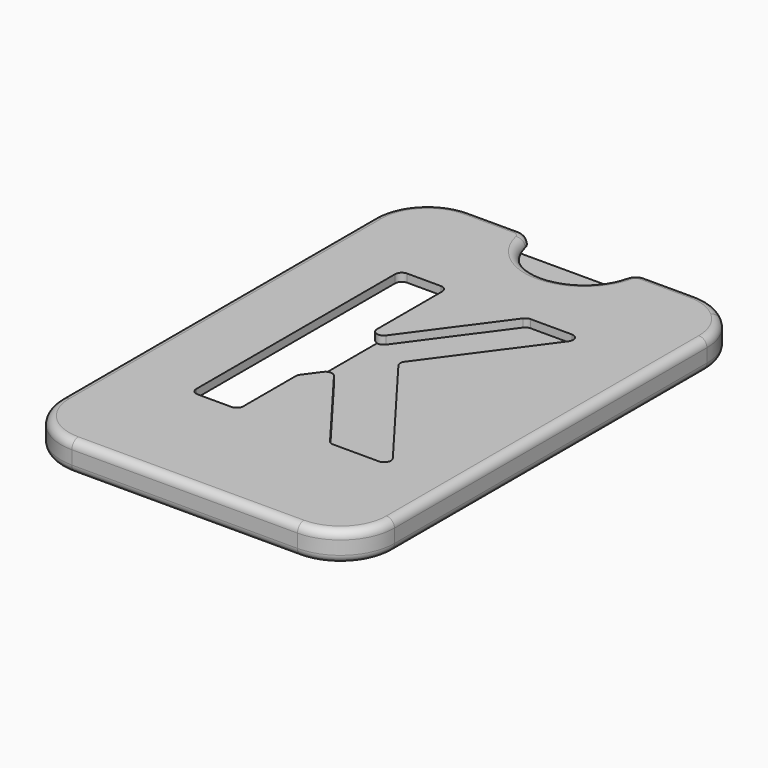
from build123d import *

# Parameters (mm, degrees)
F1_DEPTH = 2.794
F2_DEPTH = 1.27
F4_DEPTH = 2.54
F6_DEPTH = 2.54
F8_DEPTH = 2.54
F9_R     = 2.54
F10_R    = 1.52399
F11_R    = 1.27
F12_R    = 1.26999


# Not quite as in the source:
# - a fillet or chamfer is up to 0.001 mm smaller than in the source, because OpenCascade refuses the exact size


with BuildPart() as f1:
    # F0 (on Top) → F1 (new body, symmetric)
    with BuildSketch(Plane.XY):
        with BuildLine():
            Line((13.4556421247, 40.506048555), (-29.0893578753, 40.506048555))
            ThreePointArc((-29.0893578753, 40.506048555), (-32.6881934203, 39.8473107196), (-35.8203578753, 37.9565175945))
            Line((-35.8203578753, 37.9565175945), (-35.8203578753, 30.346048555))
            ThreePointArc((-35.8203578753, 30.346048555), (-33.8488936195, 35.1055842992), (-29.0893578753, 37.077048555))
            Line((-29.0893578753, 37.077048555), (13.4556421247, 37.077048555))
            ThreePointArc((13.4556421247, 37.077048555), (18.2151778689, 35.1055842992), (20.1866421247, 30.346048555))
            Line((20.1866421247, 30.346048555), (20.1866421247, 37.9565175945))
            ThreePointArc((20.1866421247, 37.9565175945), (17.0544776697, 39.8473107196), (13.4556421247, 40.506048555))
        make_face()
        with BuildLine():
            ThreePointArc((-29.0893578753, 37.077048555), (-33.8488936195, 35.1055842992), (-35.8203578753, 30.346048555))
            Line((-35.8203578753, 30.346048555), (-35.8203578753, -43.313951445))
            ThreePointArc((-35.8203578753, -43.313951445), (-33.8488936195, -48.0734871891), (-29.0893578753, -50.044951445))
            Line((-29.0893578753, -50.044951445), (13.4556421247, -50.044951445))
            ThreePointArc((13.4556421247, -50.044951445), (18.2151778689, -48.0734871891), (20.1866421247, -43.313951445))
            Line((20.1866421247, -43.313951445), (20.1866421247, 30.346048555))
            ThreePointArc((20.1866421247, 30.346048555), (18.2151778689, 35.1055842992), (13.4556421247, 37.077048555))
            Line((13.4556421247, 37.077048555), (-29.0893578753, 37.077048555))
        make_face()
        with BuildLine():
            Line((-35.8203578753, 30.346048555), (-35.8203578753, 37.9565175945))
            ThreePointArc((-35.8203578753, 37.9565175945), (-38.3525257999, 34.5196944432), (-39.2493578753, 30.346048555))
            Line((-39.2493578753, 30.346048555), (-39.2493578753, -43.313951445))
            ThreePointArc((-39.2493578753, -43.313951445), (-36.2735627721, -50.4981563418), (-29.0893578753, -53.473951445))
            Line((-29.0893578753, -53.473951445), (13.4556421247, -53.473951445))
            ThreePointArc((13.4556421247, -53.473951445), (20.6398470216, -50.4981563418), (23.6156421247, -43.313951445))
            Line((23.6156421247, -43.313951445), (23.6156421247, 30.346048555))
            ThreePointArc((23.6156421247, 30.346048555), (22.7188100493, 34.5196944432), (20.1866421247, 37.9565175945))
            Line((20.1866421247, 37.9565175945), (20.1866421247, 30.346048555))
            Line((20.1866421247, 30.346048555), (20.1866421247, -43.313951445))
            ThreePointArc((20.1866421247, -43.313951445), (18.2151778689, -48.0734871891), (13.4556421247, -50.044951445))
            Line((13.4556421247, -50.044951445), (-29.0893578753, -50.044951445))
            ThreePointArc((-29.0893578753, -50.044951445), (-33.8488936195, -48.0734871891), (-35.8203578753, -43.313951445))
            Line((-35.8203578753, -43.313951445), (-35.8203578753, 30.346048555))
        make_face()
    extrude(amount=F1_DEPTH, both=True)

    # F0 (on Top) → F2 (cut, symmetric)
    with BuildSketch(Plane.XY):
        with BuildLine():
            Line((13.4556421247, 40.506048555), (-29.0893578753, 40.506048555))
            ThreePointArc((-29.0893578753, 40.506048555), (-32.6881934203, 39.8473107196), (-35.8203578753, 37.9565175945))
            Line((-35.8203578753, 37.9565175945), (-35.8203578753, 30.346048555))
            ThreePointArc((-35.8203578753, 30.346048555), (-33.8488936195, 35.1055842992), (-29.0893578753, 37.077048555))
            Line((-29.0893578753, 37.077048555), (13.4556421247, 37.077048555))
            ThreePointArc((13.4556421247, 37.077048555), (18.2151778689, 35.1055842992), (20.1866421247, 30.346048555))
            Line((20.1866421247, 30.346048555), (20.1866421247, 37.9565175945))
            ThreePointArc((20.1866421247, 37.9565175945), (17.0544776697, 39.8473107196), (13.4556421247, 40.506048555))
        make_face()
        with BuildLine():
            ThreePointArc((-29.0893578753, 37.077048555), (-33.8488936195, 35.1055842992), (-35.8203578753, 30.346048555))
            Line((-35.8203578753, 30.346048555), (-35.8203578753, -43.313951445))
            ThreePointArc((-35.8203578753, -43.313951445), (-33.8488936195, -48.0734871891), (-29.0893578753, -50.044951445))
            Line((-29.0893578753, -50.044951445), (13.4556421247, -50.044951445))
            ThreePointArc((13.4556421247, -50.044951445), (18.2151778689, -48.0734871891), (20.1866421247, -43.313951445))
            Line((20.1866421247, -43.313951445), (20.1866421247, 30.346048555))
            ThreePointArc((20.1866421247, 30.346048555), (18.2151778689, 35.1055842992), (13.4556421247, 37.077048555))
            Line((13.4556421247, 37.077048555), (-29.0893578753, 37.077048555))
        make_face()
    extrude(amount=F2_DEPTH, both=True, mode=Mode.SUBTRACT)

    # F3 (on face) → F4 (cut)
    with BuildSketch(Plane.XY.offset(2.794)):
        Polygon((-16.199497506, 18.9658571035), (-25.0740814954, 18.9658571035), (-25.0740814954, -30.413236469), (-16.199497506, -30.413236469), (-16.199497506, -16.4083634515), (-12.8775097826, -11.8783802343), (1.1254162528, -30.413236469), (12.8968711942, -30.413236469), (-7.0793794499, -3.9718389452), (9.7415978089, 18.9658571035), (-1.1809705757, 18.9658571035), (-16.199497506, -1.5139521565), align=None)
    extrude(amount=-F4_DEPTH, mode=Mode.SUBTRACT)

    # F5 (on face) → F6 (cut)
    with BuildSketch(Plane(origin=(0, 0, -2.794), x_dir=(1, 0, 0), z_dir=(0, 0, -1))):
        with BuildLine():
            Line((-29.1631240398, 40.1679472998), (-29.1631240398, -27.4539431557))
            ThreePointArc((-29.1631240398, -27.4539431557), (-23.7097460777, -32.9073211178), (-18.2563681155, -27.4539431557))
            Line((-18.2563681155, -27.4539431557), (-18.2563681155, 40.1679472998))
            ThreePointArc((-18.2563681155, 40.1679472998), (-23.7097460777, 45.6213252619), (-29.1631240398, 40.1679472998))
        make_face()
        with BuildLine():
            ThreePointArc((-5.0461939536, -35.2972820401), (-3.9444430731, -34.1955311596), (-5.0461939536, -33.0937802792))
            Line((-5.0461939536, -33.0937802792), (-10.8487373218, -33.0937802792))
            ThreePointArc((-10.8487373218, -33.0937802792), (-11.9504882023, -34.1955311596), (-10.8487373218, -35.2972820401))
            Line((-10.8487373218, -35.2972820401), (-5.0461939536, -35.2972820401))
        make_face()
    extrude(amount=-F6_DEPTH, mode=Mode.SUBTRACT)

    # F7 (on face) → F8 (cut)
    with BuildSketch(Plane.XY.offset(2.794)):
        with BuildLine():
            Line((1.8508417322, 40.506048555), (-17.466821873, 40.506048555))
            ThreePointArc((-17.466821873, 40.506048555), (-7.8079900704, 31.0812084526), (1.8508417322, 40.506048555))
        make_face()
    extrude(amount=-F8_DEPTH, mode=Mode.SUBTRACT)

    # F9
    f9_edges = [f1.edges().sort_by_distance(p)[0] for p in [
        (1.850842, 40.506049, 2.032),
        (-17.466822, 40.506049, 2.032),
    ]]
    fillet(f9_edges, radius=F9_R)

    # F10 (radius 1.524 in the source; OpenCascade refuses exactly that, so slightly less here)
    f10_edges = [f1.edges().sort_by_distance(p)[0] for p in [
        (-39.249358, -6.483951, 2.794),
        (-39.249358, -6.483951, -2.794),
        (-29.163124, -6.357002, -2.794),
    ]]
    fillet(f10_edges, radius=F10_R)

    # F11
    f11_edges = [f1.edges().sort_by_distance(p)[0] for p in [
        (9.741598, 18.965857, 2.032),
        (-1.180971, 18.965857, 2.032),
        (-16.199498, 18.965857, 2.032),
        (-16.199498, -1.513952, 2.032),
        (-7.079379, -3.971839, 2.032),
        (12.896871, -30.413236, 2.032),
        (1.125416, -30.413236, 2.032),
        (-12.87751, -11.87838, 2.032),
        (-16.199498, -16.408363, 2.032),
        (-16.199498, -30.413236, 2.032),
        (-25.074081, -30.413236, 2.032),
        (-25.074081, 18.965857, 2.032),
    ]]
    fillet(f11_edges, radius=F11_R)

    # F12 (radius 1.27 in the source; OpenCascade refuses exactly that, so slightly less here)
    f12_edges = [f1.edges().sort_by_distance(p)[0] for p in [
        (-35.820358, -2.678717, 1.27),
        (-35.820358, -2.678717, -1.27),
    ]]
    fillet(f12_edges, radius=F12_R)


solid = f1.part
